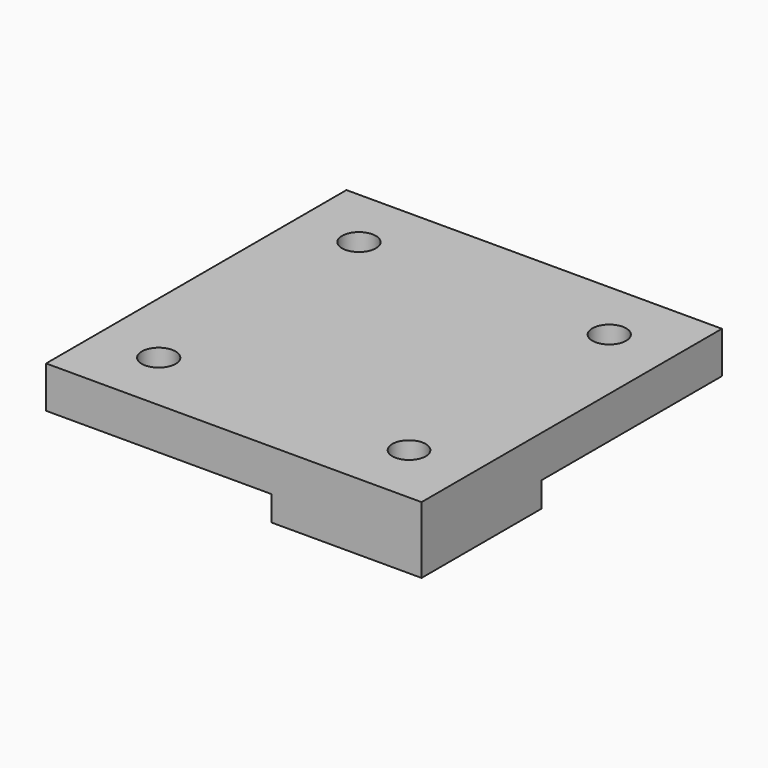
from build123d import *

# Parameters (mm, degrees)
F0_W     = 12
F0_H     = 15
F0_W_2   = 3
F1_DEPTH = 5
F2_DEPTH = 3
F3_W     = 15
F3_H     = 15
F3_R     = 2
F4_DEPTH = 8
F0_W_3   = 15
F0_R     = 2.025
F5_DEPTH = 5


# Not quite as in the source:
# - a feature names something its author has since deleted; it is built from what else it names


with BuildPart() as f1:
    # F0 (on Top) → F1 (new body)
    with BuildSketch(Plane.XY):
        with Locations((-9, -7.5)):
            Rectangle(F0_W, F0_H)
        with Locations((-1.5, -7.5)):
            Rectangle(F0_W_2, F0_H)
        Polygon((-3, 3), (-3, 0), (0, 0), (15, 0), (15, 3), align=None)
    extrude(amount=F1_DEPTH)

    # F0 (on Top) → F2 (join)
    with BuildSketch(Plane.XY):
        with Locations((-1.5, -7.5)):
            Rectangle(F0_W_2, F0_H)
        Polygon((-3, 3), (-3, 0), (0, 0), (15, 0), (15, 3), align=None)
    extrude(amount=-F2_DEPTH)

    # F3 (on face) → F4 (join)
    with BuildSketch(Plane(origin=(0, 0, -3), x_dir=(1, 0, 0), z_dir=(0, 0, -1))):
        with Locations((7.5, 7.5)):
            Rectangle(F3_W, F3_H)
        with Locations((7.5, 7.5)):
            Circle(F3_R, mode=Mode.SUBTRACT)
    extrude(amount=-F4_DEPTH)

    # F0 (on Top) → F5 (join)
    with BuildSketch(Plane.XY):
        with Locations((-22.5, -7.5)):
            Rectangle(F0_W_3, F0_H)
        with Locations((-22.5, -7.5)):
            Circle(F0_R, mode=Mode.SUBTRACT)
        with Locations((-22.5, 7.5)):
            Rectangle(F0_W_3, F0_H)
        Polygon((0, 15), (-15, 15), (-15, 0), (-3, 0), (-3, 3), (15, 3), (15, 15), align=None)
        with Locations((-7.5, 22.5)):
            Rectangle(F0_W_3, F0_H)
        with Locations((7.5, 22.5)):
            Rectangle(F0_W_3, F0_H)
        with Locations((7.5, 22.5)):
            Circle(F0_R, mode=Mode.SUBTRACT)
        with Locations((-22.5, 22.5)):
            Rectangle(F0_W_3, F0_H)
        with Locations((-22.5, 22.5)):
            Circle(F0_R, mode=Mode.SUBTRACT)
    extrude(amount=F5_DEPTH)


solid = f1.part
